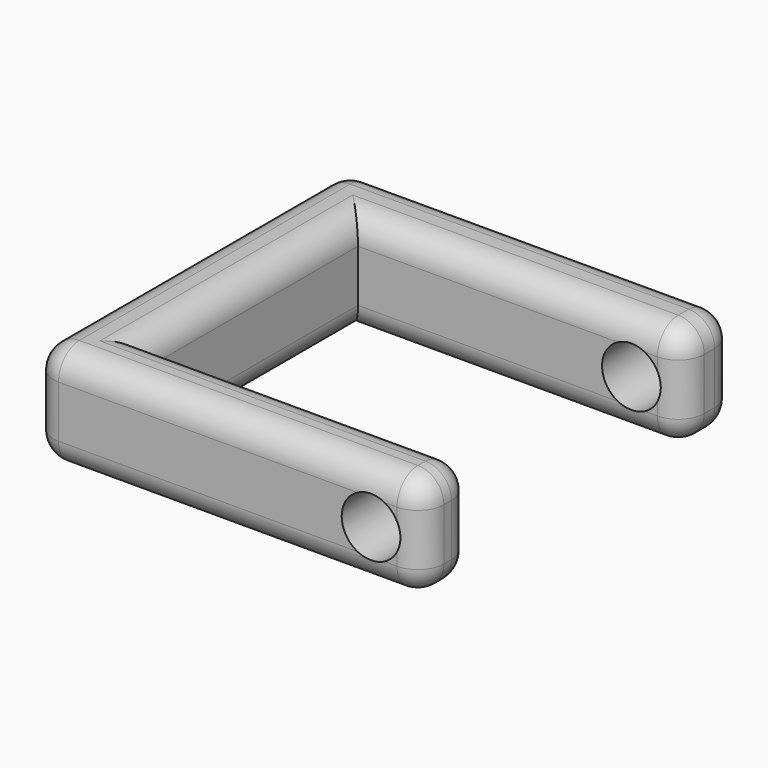
from build123d import *

# Parameters (mm, degrees)
F1_DEPTH      = 20.32
F2_R          = 5.715
F3_DEPTH      = 863.6
F4_T1_DEPTH   = 66.04
F4_T3_DEPTH   = 58.42
F4_T5_DEPTH   = 51.4949167535
F4_T7_DEPTH   = 66.04
F4_T9_DEPTH   = 10.16
F4_T11_DEPTH  = 2.54
F4_T13_DEPTH  = 1.8450832465
F4_S17_W      = 5.08
F4_S17_H      = 5.08
F4_T18_DEPTH  = 5.08
F4_S23_W      = 5.08
F4_S23_H      = 5.08
F4_T24_DEPTH  = 5.08
F4_S29_W      = 5.08
F4_S29_H      = 5.08
F4_T30_DEPTH  = 5.08
F4_S35_W      = 5.08
F4_S35_H      = 5.08
F4_T36_DEPTH  = 5.08
F4_S41_W      = 5.08
F4_S41_H      = 5.08
F4_T42_DEPTH  = 5.08
F4_S47_W      = 5.08
F4_S47_H      = 5.08
F4_T48_DEPTH  = 5.08
F4_S53_W      = 5.08
F4_S53_H      = 5.08
F4_T54_DEPTH  = 5.08
F4_S59_W      = 5.08
F4_S59_H      = 5.08
F4_T60_DEPTH  = 5.08
F4_S65_W      = 5.08
F4_S65_H      = 5.08
F4_T66_DEPTH  = 5.08
F4_S71_W      = 5.08
F4_S71_H      = 5.08
F4_T72_DEPTH  = 5.08
F4_S77_W      = 5.08
F4_S77_H      = 5.08
F4_T78_DEPTH  = 5.08
F4_S83_W      = 5.08
F4_S83_H      = 5.08
F4_T84_DEPTH  = 5.08
F4_T91_DEPTH  = 64.1949167535
F4_T95_DEPTH  = 71.12
F4_T102_DEPTH = 64.1949167535
F4_T106_DEPTH = 71.12
F4_T113_DEPTH = 71.12
F4_T117_DEPTH = 64.1949167535
F4_T124_DEPTH = 71.12
F4_T128_DEPTH = 64.1949167535


# Not quite as in the source:
# - a fillet or chamfer that OpenCascade refuses, or shapes differently, is made with other operations: its cross-section is extruded or revolved along the edge and cut away or added


with BuildPart() as f1:
    # F0 (on Top) → F1 (new body)
    with BuildSketch(Plane.XY):
        Polygon((-76.2, 0), (0, 0), (0, 12.0050832465), (-63.5, 12.0050832465), (-63.5, 63.5), (0, 63.5), (0, 76.2), (-76.2, 76.2), align=None)
    extrude(amount=F1_DEPTH)

    # F2 (on face) → F3 (cut)
    with BuildSketch(Plane.XZ):
        with Locations((-10.16, 10.16)):
            Circle(F2_R)
    extrude(amount=-F3_DEPTH, mode=Mode.SUBTRACT)

    # F4: fillet of radius 5.08 on 22 edges, made by hand

    # F4_s2 → F4_t1 (cut)
    with BuildSketch(Plane.YZ.offset(-71.12)):
        with BuildLine():
            ThreePointArc((71.12, 0), (74.7121024484, 1.4878975516), (76.2, 5.08))
            Line((76.2, 5.08), (76.2, 0))
            Line((76.2, 0), (71.12, 0))
        make_face()
        with BuildLine():
            ThreePointArc((71.12, 20.32), (74.7121024484, 18.8321024484), (76.2, 15.24))
            Line((76.2, 15.24), (76.2, 20.32))
            Line((76.2, 20.32), (71.12, 20.32))
        make_face()
        with BuildLine():
            ThreePointArc((0, 5.08), (1.4878975516, 1.4878975516), (5.08, 0))
            Line((5.08, 0), (0, 0))
            Line((0, 0), (0, 5.08))
        make_face()
        with BuildLine():
            ThreePointArc((0, 15.24), (1.4878975516, 18.8321024484), (5.08, 20.32))
            Line((5.08, 20.32), (0, 20.32))
            Line((0, 20.32), (0, 15.24))
        make_face()
    extrude(amount=F4_T1_DEPTH, mode=Mode.SUBTRACT)

    # F4_s4 → F4_t3 (cut)
    with BuildSketch(Plane.YZ.offset(-63.5)):
        with BuildLine():
            ThreePointArc((68.58, 0), (64.9878975516, 1.4878975516), (63.5, 5.08))
            Line((63.5, 5.08), (63.5, 0))
            Line((63.5, 0), (68.58, 0))
        make_face()
        with BuildLine():
            ThreePointArc((68.58, 20.32), (64.9878975516, 18.8321024484), (63.5, 15.24))
            Line((63.5, 15.24), (63.5, 20.32))
            Line((63.5, 20.32), (68.58, 20.32))
        make_face()
        with BuildLine():
            ThreePointArc((6.9250832465, 0), (10.5171856949, 1.4878975516), (12.0050832465, 5.08))
            Line((12.0050832465, 5.08), (12.0050832465, 0))
            Line((12.0050832465, 0), (6.9250832465, 0))
        make_face()
        with BuildLine():
            ThreePointArc((6.9250832465, 20.32), (10.5171856949, 18.8321024484), (12.0050832465, 15.24))
            Line((12.0050832465, 15.24), (12.0050832465, 20.32))
            Line((12.0050832465, 20.32), (6.9250832465, 20.32))
        make_face()
    extrude(amount=F4_T3_DEPTH, mode=Mode.SUBTRACT)

    # F4_s6 → F4_t5 (cut)
    with BuildSketch(Plane.XZ.offset(-63.5)):
        with BuildLine():
            ThreePointArc((-68.58, 20.32), (-64.9878975516, 18.8321024484), (-63.5, 15.24))
            Line((-63.5, 15.24), (-63.5, 20.32))
            Line((-63.5, 20.32), (-68.58, 20.32))
        make_face()
        with BuildLine():
            ThreePointArc((-68.58, 0), (-64.9878975516, 1.4878975516), (-63.5, 5.08))
            Line((-63.5, 5.08), (-63.5, 0))
            Line((-63.5, 0), (-68.58, 0))
        make_face()
    extrude(amount=F4_T5_DEPTH, mode=Mode.SUBTRACT)

    # F4_s8 → F4_t7 (cut)
    with BuildSketch(Plane.XZ.offset(-71.12)):
        with BuildLine():
            ThreePointArc((-76.2, 15.24), (-74.7121024484, 18.8321024484), (-71.12, 20.32))
            Line((-71.12, 20.32), (-76.2, 20.32))
            Line((-76.2, 20.32), (-76.2, 15.24))
        make_face()
        with BuildLine():
            ThreePointArc((-76.2, 5.08), (-74.7121024484, 1.4878975516), (-71.12, 0))
            Line((-71.12, 0), (-76.2, 0))
            Line((-76.2, 0), (-76.2, 5.08))
        make_face()
    extrude(amount=F4_T7_DEPTH, mode=Mode.SUBTRACT)

    # F4_s10 → F4_t9 (cut)
    with BuildSketch(Plane.XY.offset(5.08)):
        with BuildLine():
            ThreePointArc((-76.2, 71.12), (-74.7121024484, 74.7121024484), (-71.12, 76.2))
            Line((-71.12, 76.2), (-76.2, 76.2))
            Line((-76.2, 76.2), (-76.2, 71.12))
        make_face()
        with BuildLine():
            ThreePointArc((-71.12, 0), (-74.7121024484, 1.4878975516), (-76.2, 5.08))
            Line((-76.2, 5.08), (-76.2, 0))
            Line((-76.2, 0), (-71.12, 0))
        make_face()
        with BuildLine():
            ThreePointArc((-5.08, 63.5), (-1.4878975516, 64.9878975516), (0, 68.58))
            Line((0, 68.58), (0, 63.5))
            Line((0, 63.5), (-5.08, 63.5))
        make_face()
        with BuildLine():
            ThreePointArc((-5.08, 76.2), (-1.4878975516, 74.7121024484), (0, 71.12))
            Line((0, 71.12), (0, 76.2))
            Line((0, 76.2), (-5.08, 76.2))
        make_face()
        with BuildLine():
            ThreePointArc((-5.08, 0), (-1.4878975516, 1.4878975516), (0, 5.08))
            Line((0, 5.08), (0, 0))
            Line((0, 0), (-5.08, 0))
        make_face()
        with BuildLine():
            ThreePointArc((0, 6.9250832465), (-1.4878975516, 10.5171856949), (-5.08, 12.0050832465))
            Line((-5.08, 12.0050832465), (0, 12.0050832465))
            Line((0, 12.0050832465), (0, 6.9250832465))
        make_face()
    extrude(amount=F4_T9_DEPTH, mode=Mode.SUBTRACT)

    # F4_s12 → F4_t11 (cut)
    with BuildSketch(Plane.XZ.offset(-71.12)):
        with BuildLine():
            ThreePointArc((-5.08, 0), (-1.4878975516, 1.4878975516), (0, 5.08))
            Line((0, 5.08), (0, 0))
            Line((0, 0), (-5.08, 0))
        make_face()
        with BuildLine():
            ThreePointArc((-5.08, 20.32), (-1.4878975516, 18.8321024484), (0, 15.24))
            Line((0, 15.24), (0, 20.32))
            Line((0, 20.32), (-5.08, 20.32))
        make_face()
    extrude(amount=F4_T11_DEPTH, mode=Mode.SUBTRACT)

    # F4_s14 → F4_t13 (cut)
    with BuildSketch(Plane.XZ.offset(-6.9250832465)):
        with BuildLine():
            ThreePointArc((-5.08, 0), (-1.4878975516, 1.4878975516), (0, 5.08))
            Line((0, 5.08), (0, 0))
            Line((0, 0), (-5.08, 0))
        make_face()
        with BuildLine():
            ThreePointArc((-5.08, 20.32), (-1.4878975516, 18.8321024484), (0, 15.24))
            Line((0, 15.24), (0, 20.32))
            Line((0, 20.32), (-5.08, 20.32))
        make_face()
    extrude(amount=F4_T13_DEPTH, mode=Mode.SUBTRACT)


with BuildPart() as f4_tool16:
    # F4_s17 → F4_t18 (new body)
    with BuildSketch(Plane.XY.offset(5.08)):
        with Locations((-2.54, 73.66)):
            Rectangle(F4_S17_W, F4_S17_H)
    extrude(amount=-F4_T18_DEPTH)

    # F4_s19 → F4_t20 (revolve, cut)
    with BuildSketch(Plane(origin=(-5.08, 71.12, 5.08), x_dir=(-0.7071067812, -0.7071067812, 0), z_dir=(0.7071067812, -0.7071067812, 0))):
        with BuildLine():
            ThreePointArc((0, -5.08), (5.08, 0), (0, 5.08))
            Line((0, 5.08), (0, -5.08))
        make_face()
    revolve(axis=Axis((-5.08, 71.12, 5.08), (0, 0, -1)), mode=Mode.SUBTRACT)


with BuildPart() as f1_1:
    add(f1.part)

    # F4_t15: cut F4_tool16
    add(f4_tool16.part, mode=Mode.SUBTRACT)


with BuildPart() as f4_tool22:
    # F4_s23 → F4_t24 (new body)
    with BuildSketch(Plane.YZ.offset(-71.12)):
        with Locations((73.66, 2.54)):
            Rectangle(F4_S23_W, F4_S23_H)
    extrude(amount=-F4_T24_DEPTH)

    # F4_s25 → F4_t26 (revolve, cut)
    with BuildSketch(Plane(origin=(-71.12, 71.12, 5.08), x_dir=(0, -0.7071067812, 0.7071067812), z_dir=(0, -0.7071067812, -0.7071067812))):
        with BuildLine():
            ThreePointArc((0, -5.08), (5.08, 0), (0, 5.08))
            Line((0, 5.08), (0, -5.08))
        make_face()
    revolve(axis=Axis((-71.12, 71.12, 5.08), (-1, 0, 0)), mode=Mode.SUBTRACT)


with BuildPart() as f1_2:
    add(f1_1.part)

    # F4_t21: cut F4_tool22
    add(f4_tool22.part, mode=Mode.SUBTRACT)


with BuildPart() as f4_tool28:
    # F4_s29 → F4_t30 (new body)
    with BuildSketch(Plane.XZ.offset(-68.58)):
        with Locations((-2.54, 2.54)):
            Rectangle(F4_S29_W, F4_S29_H)
    extrude(amount=F4_T30_DEPTH)

    # F4_s31 → F4_t32 (revolve, cut)
    with BuildSketch(Plane(origin=(-5.08, 68.58, 5.08), x_dir=(-0.7071067812, 0, 0.7071067812), z_dir=(0.7071067812, 0, 0.7071067812))):
        with BuildLine():
            ThreePointArc((0, -5.08), (5.08, 0), (0, 5.08))
            Line((0, 5.08), (0, -5.08))
        make_face()
    revolve(axis=Axis((-5.08, 68.58, 5.08), (0, -1, 0)), mode=Mode.SUBTRACT)


with BuildPart() as f1_3:
    add(f1_2.part)

    # F4_t27: cut F4_tool28
    add(f4_tool28.part, mode=Mode.SUBTRACT)


with BuildPart() as f4_tool34:
    # F4_s35 → F4_t36 (new body)
    with BuildSketch(Plane.XZ.offset(-68.58)):
        with Locations((-2.54, 17.78)):
            Rectangle(F4_S35_W, F4_S35_H)
    extrude(amount=F4_T36_DEPTH)

    # F4_s37 → F4_t38 (revolve, cut)
    with BuildSketch(Plane(origin=(-5.08, 68.58, 15.24), x_dir=(-0.7071067812, 0, -0.7071067812), z_dir=(-0.7071067812, 0, 0.7071067812))):
        with BuildLine():
            ThreePointArc((0, -5.08), (5.08, 0), (0, 5.08))
            Line((0, 5.08), (0, -5.08))
        make_face()
    revolve(axis=Axis((-5.08, 68.58, 15.24), (0, -1, 0)), mode=Mode.SUBTRACT)


with BuildPart() as f1_4:
    add(f1_3.part)

    # F4_t33: cut F4_tool34
    add(f4_tool34.part, mode=Mode.SUBTRACT)


with BuildPart() as f4_tool40:
    # F4_s41 → F4_t42 (new body)
    with BuildSketch(Plane.YZ.offset(-5.08)):
        with Locations((73.66, 17.78)):
            Rectangle(F4_S41_W, F4_S41_H)
    extrude(amount=F4_T42_DEPTH)

    # F4_s43 → F4_t44 (revolve, cut)
    with BuildSketch(Plane(origin=(-5.08, 71.12, 15.24), x_dir=(0, -0.7071067812, -0.7071067812), z_dir=(0, -0.7071067812, 0.7071067812))):
        with BuildLine():
            ThreePointArc((0, -5.08), (5.08, 0), (0, 5.08))
            Line((0, 5.08), (0, -5.08))
        make_face()
    revolve(axis=Axis((-5.08, 71.12, 15.24), (1, 0, 0)), mode=Mode.SUBTRACT)


with BuildPart() as f1_5:
    add(f1_4.part)

    # F4_t39: cut F4_tool40
    add(f4_tool40.part, mode=Mode.SUBTRACT)


with BuildPart() as f4_tool46:
    # F4_s47 → F4_t48 (new body)
    with BuildSketch(Plane.YZ.offset(-71.12)):
        with Locations((73.66, 17.78)):
            Rectangle(F4_S47_W, F4_S47_H)
    extrude(amount=-F4_T48_DEPTH)

    # F4_s49 → F4_t50 (revolve, cut)
    with BuildSketch(Plane(origin=(-71.12, 71.12, 15.24), x_dir=(0, -0.7071067812, -0.7071067812), z_dir=(0, 0.7071067812, -0.7071067812))):
        with BuildLine():
            ThreePointArc((0, -5.08), (5.08, 0), (0, 5.08))
            Line((0, 5.08), (0, -5.08))
        make_face()
    revolve(axis=Axis((-71.12, 71.12, 15.24), (-1, 0, 0)), mode=Mode.SUBTRACT)


with BuildPart() as f1_6:
    add(f1_5.part)

    # F4_t45: cut F4_tool46
    add(f4_tool46.part, mode=Mode.SUBTRACT)


with BuildPart() as f4_tool52:
    # F4_s53 → F4_t54 (new body)
    with BuildSketch(Plane.XZ.offset(-5.08)):
        with Locations((-73.66, 17.78)):
            Rectangle(F4_S53_W, F4_S53_H)
    extrude(amount=F4_T54_DEPTH)

    # F4_s55 → F4_t56 (revolve, cut)
    with BuildSketch(Plane(origin=(-71.12, 5.08, 15.24), x_dir=(0.7071067812, 0, -0.7071067812), z_dir=(-0.7071067812, 0, -0.7071067812))):
        with BuildLine():
            ThreePointArc((0, -5.08), (5.08, 0), (0, 5.08))
            Line((0, 5.08), (0, -5.08))
        make_face()
    revolve(axis=Axis((-71.12, 5.08, 15.24), (0, -1, 0)), mode=Mode.SUBTRACT)


with BuildPart() as f1_7:
    add(f1_6.part)

    # F4_t51: cut F4_tool52
    add(f4_tool52.part, mode=Mode.SUBTRACT)


with BuildPart() as f4_tool58:
    # F4_s59 → F4_t60 (new body)
    with BuildSketch(Plane.XZ.offset(-5.08)):
        with Locations((-73.66, 2.54)):
            Rectangle(F4_S59_W, F4_S59_H)
    extrude(amount=F4_T60_DEPTH)

    # F4_s61 → F4_t62 (revolve, cut)
    with BuildSketch(Plane(origin=(-71.12, 5.08, 5.08), x_dir=(0.7071067812, 0, 0.7071067812), z_dir=(0.7071067812, 0, -0.7071067812))):
        with BuildLine():
            ThreePointArc((0, -5.08), (5.08, 0), (0, 5.08))
            Line((0, 5.08), (0, -5.08))
        make_face()
    revolve(axis=Axis((-71.12, 5.08, 5.08), (0, -1, 0)), mode=Mode.SUBTRACT)


with BuildPart() as f1_8:
    add(f1_7.part)

    # F4_t57: cut F4_tool58
    add(f4_tool58.part, mode=Mode.SUBTRACT)


with BuildPart() as f4_tool64:
    # F4_s65 → F4_t66 (new body)
    with BuildSketch(Plane.XZ.offset(-5.08)):
        with Locations((-2.54, 2.54)):
            Rectangle(F4_S65_W, F4_S65_H)
    extrude(amount=F4_T66_DEPTH)

    # F4_s67 → F4_t68 (revolve, cut)
    with BuildSketch(Plane(origin=(-5.08, 5.08, 5.08), x_dir=(-0.7071067812, 0, 0.7071067812), z_dir=(0.7071067812, 0, 0.7071067812))):
        with BuildLine():
            ThreePointArc((0, -5.08), (5.08, 0), (0, 5.08))
            Line((0, 5.08), (0, -5.08))
        make_face()
    revolve(axis=Axis((-5.08, 5.08, 5.08), (0, -1, 0)), mode=Mode.SUBTRACT)


with BuildPart() as f1_9:
    add(f1_8.part)

    # F4_t63: cut F4_tool64
    add(f4_tool64.part, mode=Mode.SUBTRACT)


with BuildPart() as f4_tool70:
    # F4_s71 → F4_t72 (new body)
    with BuildSketch(Plane.XZ.offset(-5.08)):
        with Locations((-2.54, 17.78)):
            Rectangle(F4_S71_W, F4_S71_H)
    extrude(amount=F4_T72_DEPTH)

    # F4_s73 → F4_t74 (revolve, cut)
    with BuildSketch(Plane(origin=(-5.08, 5.08, 15.24), x_dir=(-0.7071067812, 0, -0.7071067812), z_dir=(-0.7071067812, 0, 0.7071067812))):
        with BuildLine():
            ThreePointArc((0, -5.08), (5.08, 0), (0, 5.08))
            Line((0, 5.08), (0, -5.08))
        make_face()
    revolve(axis=Axis((-5.08, 5.08, 15.24), (0, -1, 0)), mode=Mode.SUBTRACT)


with BuildPart() as f1_10:
    add(f1_9.part)

    # F4_t69: cut F4_tool70
    add(f4_tool70.part, mode=Mode.SUBTRACT)


with BuildPart() as f4_tool76:
    # F4_s77 → F4_t78 (new body)
    with BuildSketch(Plane.XY.offset(5.08)):
        with Locations((-2.54, 9.4650832465)):
            Rectangle(F4_S77_W, F4_S77_H)
    extrude(amount=-F4_T78_DEPTH)

    # F4_s79 → F4_t80 (revolve, cut)
    with BuildSketch(Plane(origin=(-5.08, 6.9250832465, 5.08), x_dir=(-0.7071067812, -0.7071067812, 0), z_dir=(0.7071067812, -0.7071067812, 0))):
        with BuildLine():
            ThreePointArc((0, -5.08), (5.08, 0), (0, 5.08))
            Line((0, 5.08), (0, -5.08))
        make_face()
    revolve(axis=Axis((-5.08, 6.9250832465, 5.08), (0, 0, -1)), mode=Mode.SUBTRACT)


with BuildPart() as f1_11:
    add(f1_10.part)

    # F4_t75: cut F4_tool76
    add(f4_tool76.part, mode=Mode.SUBTRACT)


with BuildPart() as f4_tool82:
    # F4_s83 → F4_t84 (new body)
    with BuildSketch(Plane.XY.offset(15.24)):
        with Locations((-2.54, 9.4650832465)):
            Rectangle(F4_S83_W, F4_S83_H)
    extrude(amount=F4_T84_DEPTH)

    # F4_s85 → F4_t86 (revolve, cut)
    with BuildSketch(Plane(origin=(-5.08, 6.9250832465, 15.24), x_dir=(-0.7071067812, -0.7071067812, 0), z_dir=(-0.7071067812, 0.7071067812, 0))):
        with BuildLine():
            ThreePointArc((0, -5.08), (5.08, 0), (0, 5.08))
            Line((0, 5.08), (0, -5.08))
        make_face()
    revolve(axis=Axis((-5.08, 6.9250832465, 15.24), (0, 0, 1)), mode=Mode.SUBTRACT)


with BuildPart() as f1_12:
    add(f1_11.part)

    # F4_t81: cut F4_tool82
    add(f4_tool82.part, mode=Mode.SUBTRACT)


with BuildPart() as f4_tool89:
    # F4_s90 → F4_t91 (new body)
    with BuildSketch(Plane.XZ.offset(-12.0050832465)):
        with BuildLine():
            ThreePointArc((-68.58, 0), (-64.9878975516, 1.4878975516), (-63.5, 5.08))
            Line((-63.5, 5.08), (-63.5, 0))
            Line((-63.5, 0), (-68.58, 0))
        make_face()
    extrude(amount=-F4_T91_DEPTH)

    split(bisect_by=Plane.XZ.offset(-63.5), keep=Keep.BOTTOM)


with BuildPart() as f4_tool93:
    # F4_s94 → F4_t95 (new body)
    with BuildSketch(Plane.YZ.offset(-76.2)):
        with BuildLine():
            ThreePointArc((68.58, 0), (64.9878975516, 1.4878975516), (63.5, 5.08))
            Line((63.5, 5.08), (63.5, 0))
            Line((63.5, 0), (68.58, 0))
        make_face()
    extrude(amount=F4_T95_DEPTH)

    split(bisect_by=Plane.YZ.offset(-63.5), keep=Keep.BOTTOM)


with BuildPart() as f4_tool89_1:
    add(f4_tool89.part)

    # F4_t97: intersect F4_tool93
    add(f4_tool93.part, mode=Mode.INTERSECT)


with BuildPart() as f1_13:
    add(f1_12.part)

    # F4_t87: cut F4_tool89
    add(f4_tool89_1.part, mode=Mode.SUBTRACT)


with BuildPart() as f4_tool100:
    # F4_s101 → F4_t102 (new body)
    with BuildSketch(Plane.XZ.offset(-12.0050832465)):
        with BuildLine():
            ThreePointArc((-68.58, 20.32), (-64.9878975516, 18.8321024484), (-63.5, 15.24))
            Line((-63.5, 15.24), (-63.5, 20.32))
            Line((-63.5, 20.32), (-68.58, 20.32))
        make_face()
    extrude(amount=-F4_T102_DEPTH)

    split(bisect_by=Plane.XZ.offset(-63.5), keep=Keep.BOTTOM)


with BuildPart() as f4_tool104:
    # F4_s105 → F4_t106 (new body)
    with BuildSketch(Plane.YZ.offset(-76.2)):
        with BuildLine():
            ThreePointArc((68.58, 20.32), (64.9878975516, 18.8321024484), (63.5, 15.24))
            Line((63.5, 15.24), (63.5, 20.32))
            Line((63.5, 20.32), (68.58, 20.32))
        make_face()
    extrude(amount=F4_T106_DEPTH)

    split(bisect_by=Plane.YZ.offset(-63.5), keep=Keep.BOTTOM)


with BuildPart() as f4_tool100_1:
    add(f4_tool100.part)

    # F4_t108: intersect F4_tool104
    add(f4_tool104.part, mode=Mode.INTERSECT)


with BuildPart() as f1_14:
    add(f1_13.part)

    # F4_t98: cut F4_tool100
    add(f4_tool100_1.part, mode=Mode.SUBTRACT)


with BuildPart() as f4_tool111:
    # F4_s112 → F4_t113 (new body)
    with BuildSketch(Plane.YZ.offset(-5.08)):
        with BuildLine():
            ThreePointArc((6.9250832465, 20.32), (10.5171856949, 18.8321024484), (12.0050832465, 15.24))
            Line((12.0050832465, 15.24), (12.0050832465, 20.32))
            Line((12.0050832465, 20.32), (6.9250832465, 20.32))
        make_face()
    extrude(amount=-F4_T113_DEPTH)

    split(bisect_by=Plane.YZ.offset(-63.5), keep=Keep.BOTTOM)


with BuildPart() as f4_tool115:
    # F4_s116 → F4_t117 (new body)
    with BuildSketch(Plane.XZ.offset(0.6949167535)):
        with BuildLine():
            ThreePointArc((-68.58, 20.32), (-64.9878975516, 18.8321024484), (-63.5, 15.24))
            Line((-63.5, 15.24), (-63.5, 20.32))
            Line((-63.5, 20.32), (-68.58, 20.32))
        make_face()
    extrude(amount=-F4_T117_DEPTH)

    split(bisect_by=Plane.XZ.offset(-12.0050832465), keep=Keep.TOP)


with BuildPart() as f4_tool111_1:
    add(f4_tool111.part)

    # F4_t119: intersect F4_tool115
    add(f4_tool115.part, mode=Mode.INTERSECT)


with BuildPart() as f1_15:
    add(f1_14.part)

    # F4_t109: cut F4_tool111
    add(f4_tool111_1.part, mode=Mode.SUBTRACT)


with BuildPart() as f4_tool122:
    # F4_s123 → F4_t124 (new body)
    with BuildSketch(Plane.YZ.offset(-5.08)):
        with BuildLine():
            ThreePointArc((6.9250832465, 0), (10.5171856949, 1.4878975516), (12.0050832465, 5.08))
            Line((12.0050832465, 5.08), (12.0050832465, 0))
            Line((12.0050832465, 0), (6.9250832465, 0))
        make_face()
    extrude(amount=-F4_T124_DEPTH)

    split(bisect_by=Plane.YZ.offset(-63.5), keep=Keep.BOTTOM)


with BuildPart() as f4_tool126:
    # F4_s127 → F4_t128 (new body)
    with BuildSketch(Plane.XZ.offset(0.6949167535)):
        with BuildLine():
            ThreePointArc((-68.58, 0), (-64.9878975516, 1.4878975516), (-63.5, 5.08))
            Line((-63.5, 5.08), (-63.5, 0))
            Line((-63.5, 0), (-68.58, 0))
        make_face()
    extrude(amount=-F4_T128_DEPTH)

    split(bisect_by=Plane.XZ.offset(-12.0050832465), keep=Keep.TOP)


with BuildPart() as f4_tool122_1:
    add(f4_tool122.part)

    # F4_t130: intersect F4_tool126
    add(f4_tool126.part, mode=Mode.INTERSECT)


with BuildPart() as f1_16:
    add(f1_15.part)

    # F4_t120: cut F4_tool122
    add(f4_tool122_1.part, mode=Mode.SUBTRACT)


solid = f1_16.part
